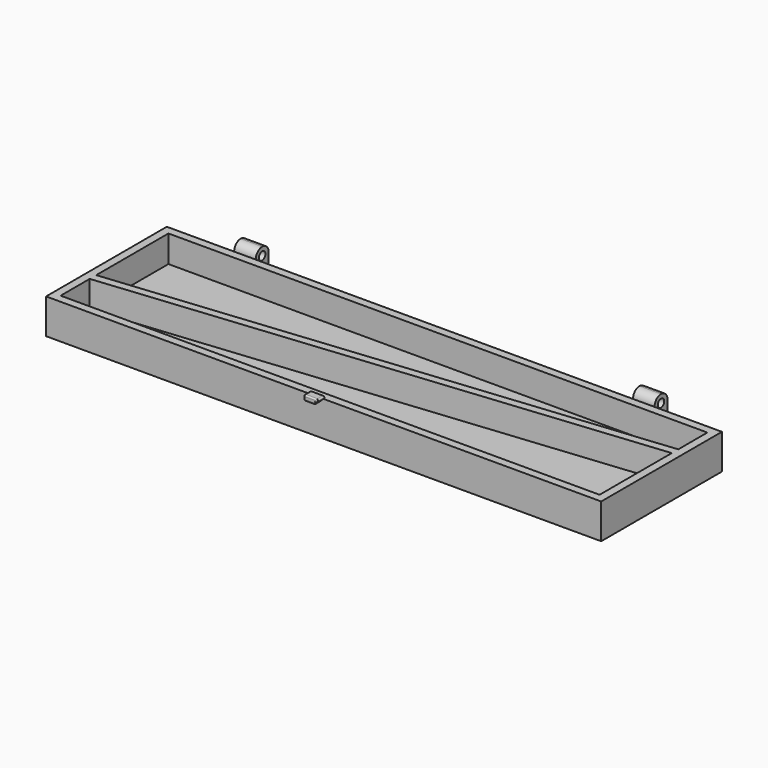
from build123d import *

# Parameters (mm, degrees)
F0_W          = 206
F0_H          = 56
F1_DEPTH      = 13
F2_T          = -3
F4_DEPTH      = 10
F5_W          = 8
F5_H          = 13
F6_DEPTH      = 6
F7_W          = 8
F7_H          = 6
F8_DEPTH      = 3
F9_R          = 2.99999
F11_D         = 3
F12_W         = 5.25
F12_H         = 1
F13_DEPTH     = 3
F14_T1_DEPTH  = 5.5
F14_T3_DEPTH  = 4.1572120132
F14_T5_DEPTH  = 3.75
F14_T7_DEPTH  = 6
F14_T9_DEPTH  = 3.25
F14_T11_DEPTH = 2.5
F14_T13_DEPTH = 1
F14_S17_W     = 0.5
F14_S17_H     = 0.5
F14_T18_DEPTH = 0.5
F14_S23_W     = 0.5
F14_S23_H     = 0.5
F14_T24_DEPTH = 0.5
F14_S29_W     = 0.5
F14_S29_H     = 0.5
F14_T30_DEPTH = 0.5
F14_T36_DEPTH = 1.6727936268


# Not quite as in the source:
# - a fillet or chamfer that OpenCascade refuses, or shapes differently, is made with other operations: its cross-section is extruded or revolved along the edge and cut away or added
# - a fillet or chamfer is up to 0.001 mm smaller than in the source, because OpenCascade refuses the exact size


with BuildPart() as f1:
    # F0 (on Top) → F1 (new body)
    with BuildSketch(Plane.XY):
        Rectangle(F0_W, F0_H)
    extrude(amount=F1_DEPTH)

    # F2
    f2_openings = [f1.faces().sort_by_distance(p)[0] for p in [
        (0, 0, 13),
    ]]
    offset(amount=F2_T, openings=f2_openings)

    # F3 (on face) → F4 (join)
    with BuildSketch(Plane.XY.offset(3)):
        Polygon((100, 11.5), (-100, -8.5), (-100, -11.5), (100, 8.5), align=None)
    extrude(amount=F4_DEPTH)

    # F5 (on face) → F6 (join)
    with BuildSketch(Plane(origin=(0, 28, 0), x_dir=(-1, 0, 0), z_dir=(0, 1, 0))):
        with Locations((-74, 6.5)):
            Rectangle(F5_W, F5_H)
        with Locations((74, 6.5)):
            Rectangle(F5_W, F5_H)
    extrude(amount=F6_DEPTH)

    # F7 (on face) → F8 (join)
    with BuildSketch(Plane.XY.offset(13)):
        with Locations((-74, 31)):
            Rectangle(F7_W, F7_H)
        with Locations((74, 31)):
            Rectangle(F7_W, F7_H)
    extrude(amount=F8_DEPTH)

    # F9 (radius 3 in the source; OpenCascade refuses exactly that, so slightly less here)
    f9_edges = [f1.edges().sort_by_distance(p)[0] for p in [
        (-74, 28, 16),
        (-74, 34, 16),
        (74, 34, 16),
        (74, 28, 16),
    ]]
    fillet(f9_edges, radius=F9_R)

    # F11 (through all)
    with Locations(Plane.YZ.offset(78)):
        with Locations((31, 13)):
            Hole(F11_D / 2)

    # F12 (on face) → F13 (join)
    with BuildSketch(Plane.XZ.offset(28)):
        Polygon((-0.75, 12.9227936268), (0.25, 13), (-5, 13), (-5, 12), (-0.75, 12), align=None)
        with Locations((-2.375, 13.5)):
            Rectangle(F12_W, F12_H)
    extrude(amount=F13_DEPTH)

    # F14: fillet of radius 0.5 on 9 edges, made by hand

    # F14_s2 → F14_t1 (cut)
    with BuildSketch(Plane.XZ.offset(26.75)):
        with BuildLine():
            ThreePointArc((0.25, 13.5), (0.1035533906, 13.8535533906), (-0.25, 14))
            Line((-0.25, 14), (0.25, 14))
            Line((0.25, 14), (0.25, 13.5))
        make_face()
    extrude(amount=F14_T1_DEPTH, mode=Mode.SUBTRACT)

    # F14_s4 → F14_t3 (cut)
    with BuildSketch(Plane.XZ.offset(28)):
        with BuildLine():
            ThreePointArc((-0.211511355, 12.9643683821), (0.1169089277, 13.1232116701), (0.25, 13.4628848053))
            Line((0.25, 13.4628848053), (0.25, 13))
            Line((0.25, 13), (-0.211511355, 12.9643683821))
        make_face()
    extrude(amount=F14_T3_DEPTH, mode=Mode.SUBTRACT)

    # F14_s6 → F14_t5 (cut)
    with BuildSketch(Plane.XZ.offset(26.75)):
        with BuildLine():
            ThreePointArc((-5, 13.5), (-4.8535533906, 13.8535533906), (-4.5, 14))
            Line((-4.5, 14), (-5, 14))
            Line((-5, 14), (-5, 13.5))
        make_face()
    extrude(amount=F14_T5_DEPTH, mode=Mode.SUBTRACT)

    # F14_s8 → F14_t7 (cut)
    with BuildSketch(Plane.YZ.offset(-4.5)):
        with BuildLine():
            ThreePointArc((-31, 13.5), (-30.8535533906, 13.8535533906), (-30.5, 14))
            Line((-30.5, 14), (-31, 14))
            Line((-31, 14), (-31, 13.5))
        make_face()
    extrude(amount=F14_T7_DEPTH, mode=Mode.SUBTRACT)

    # F14_s10 → F14_t9 (cut)
    with BuildSketch(Plane.YZ.offset(-4.5)):
        with BuildLine():
            ThreePointArc((-30.5, 12), (-30.8535533906, 12.1464466094), (-31, 12.5))
            Line((-31, 12.5), (-31, 12))
            Line((-31, 12), (-30.5, 12))
        make_face()
    extrude(amount=F14_T9_DEPTH, mode=Mode.SUBTRACT)

    # F14_s12 → F14_t11 (cut)
    with BuildSketch(Plane.XZ.offset(28)):
        with BuildLine():
            ThreePointArc((-0.75, 12.5), (-0.8964466094, 12.1464466094), (-1.25, 12))
            Line((-1.25, 12), (-0.75, 12))
            Line((-0.75, 12), (-0.75, 12.5))
        make_face()
        with BuildLine():
            ThreePointArc((-4.5, 12), (-4.8535533906, 12.1464466094), (-5, 12.5))
            Line((-5, 12.5), (-5, 12))
            Line((-5, 12), (-4.5, 12))
        make_face()
    extrude(amount=F14_T11_DEPTH, mode=Mode.SUBTRACT)

    # F14_s14 → F14_t13 (cut)
    with BuildSketch(Plane.XY.offset(12.5)):
        with BuildLine():
            ThreePointArc((-5, -30.5), (-4.8535533906, -30.8535533906), (-4.5, -31))
            Line((-4.5, -31), (-5, -31))
            Line((-5, -31), (-5, -30.5))
        make_face()
    extrude(amount=F14_T13_DEPTH, mode=Mode.SUBTRACT)


with BuildPart() as f14_tool16:
    # F14_s17 → F14_t18 (new body)
    with BuildSketch(Plane.YZ.offset(-4.5)):
        with Locations((-30.75, 13.75)):
            Rectangle(F14_S17_W, F14_S17_H)
    extrude(amount=-F14_T18_DEPTH)

    # F14_s19 → F14_t20 (revolve, cut)
    with BuildSketch(Plane(origin=(-4.5, -30.5, 13.5), x_dir=(0, 0.7071067812, -0.7071067812), z_dir=(0, 0.7071067812, 0.7071067812))):
        with BuildLine():
            ThreePointArc((0, -0.5), (0.5, 0), (0, 0.5))
            Line((0, 0.5), (0, -0.5))
        make_face()
    revolve(axis=Axis((-4.5, -30.5, 13.5), (-1, 0, 0)), mode=Mode.SUBTRACT)


with BuildPart() as f1_1:
    add(f1.part)

    # F14_t15: cut F14_tool16
    add(f14_tool16.part, mode=Mode.SUBTRACT)


with BuildPart() as f14_tool22:
    # F14_s23 → F14_t24 (new body)
    with BuildSketch(Plane.XY.offset(12.5)):
        with Locations((-4.75, -30.75)):
            Rectangle(F14_S23_W, F14_S23_H)
    extrude(amount=-F14_T24_DEPTH)

    # F14_s25 → F14_t26 (revolve, cut)
    with BuildSketch(Plane(origin=(-4.5, -30.5, 12.5), x_dir=(0.7071067812, 0.7071067812, 0), z_dir=(-0.7071067812, 0.7071067812, 0))):
        with BuildLine():
            ThreePointArc((0, -0.5), (0.5, 0), (0, 0.5))
            Line((0, 0.5), (0, -0.5))
        make_face()
    revolve(axis=Axis((-4.5, -30.5, 12.5), (0, 0, -1)), mode=Mode.SUBTRACT)


with BuildPart() as f1_2:
    add(f1_1.part)

    # F14_t21: cut F14_tool22
    add(f14_tool22.part, mode=Mode.SUBTRACT)


with BuildPart() as f14_tool28:
    # F14_s29 → F14_t30 (new body)
    with BuildSketch(Plane.YZ.offset(-1.25)):
        with Locations((-30.75, 12.25)):
            Rectangle(F14_S29_W, F14_S29_H)
    extrude(amount=F14_T30_DEPTH)

    # F14_s31 → F14_t32 (revolve, cut)
    with BuildSketch(Plane(origin=(-1.25, -30.5, 12.5), x_dir=(0, 0.7071067812, 0.7071067812), z_dir=(0, 0.7071067812, -0.7071067812))):
        with BuildLine():
            ThreePointArc((0, -0.5), (0.5, 0), (0, 0.5))
            Line((0, 0.5), (0, -0.5))
        make_face()
    revolve(axis=Axis((-1.25, -30.5, 12.5), (1, 0, 0)), mode=Mode.SUBTRACT)


with BuildPart() as f1_3:
    add(f1_2.part)

    # F14_t27: cut F14_tool28
    add(f14_tool28.part, mode=Mode.SUBTRACT)


with BuildPart() as f14_tool34:
    # F14_s35 → F14_t36 (new body)
    with BuildSketch(Plane.XY.offset(12.5)):
        with BuildLine():
            ThreePointArc((-0.75, -30.5), (-0.8964466094, -30.8535533906), (-1.25, -31))
            Line((-1.25, -31), (-0.75, -31))
            Line((-0.75, -31), (-0.75, -30.5))
        make_face()
    extrude(amount=F14_T36_DEPTH)

    split(bisect_by=Plane(origin=(-0.9962541501, 0, 12.903781237), x_dir=(0, 1, 0), z_dir=(0.07697729, 0, -0.9970328464)), keep=Keep.TOP)


with BuildPart() as f1_4:
    add(f1_3.part)

    # F14_t33: cut F14_tool34
    add(f14_tool34.part, mode=Mode.SUBTRACT)


solid = f1_4.part
